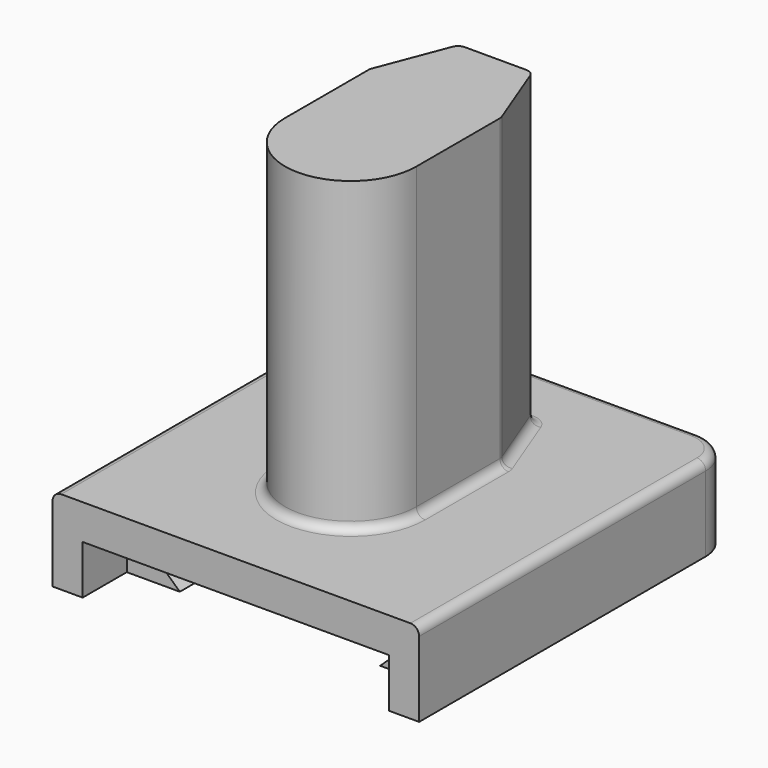
from build123d import *

# Parameters (mm, degrees)
F1_DEPTH = 2.4
F3_DEPTH = 17.61
F5_DEPTH = 2.8
F7_DEPTH = 16.06
F8_R     = 0.5


with BuildPart() as f1:
    # F0 (on Top) → F1 (new body, symmetric)
    with BuildSketch(Plane.XY):
        with BuildLine():
            ThreePointArc((10.47, 9.23), (9.8842135624, 10.6442135624), (8.47, 11.23))
            Line((8.47, 11.23), (-8.47, 11.23))
            ThreePointArc((-8.47, 11.23), (-9.8842135624, 10.6442135624), (-10.47, 9.23))
            Line((-10.47, 9.23), (-10.47, -11.23))
            Line((-10.47, -11.23), (10.47, -11.23))
            Line((10.47, -11.23), (10.47, 9.23))
        make_face()
    extrude(amount=F1_DEPTH, both=True)

    # F2 (on face) → F3 (join)
    with BuildSketch(Plane.XY.offset(2.4)):
        with BuildLine():
            ThreePointArc((-3.75, -3.025), (0, -6.775), (3.75, -3.025))
            Line((3.75, -3.025), (3.75, 3.025))
            Line((3.75, 3.025), (2.1, 7.325))
            Line((2.1, 7.325), (-2.1, 7.325))
            Line((-2.1, 7.325), (-3.75, 3.025))
            Line((-3.75, 3.025), (-3.75, -3.025))
        make_face()
    extrude(amount=F3_DEPTH)

    # F4 (on face) → F5 (cut)
    with BuildSketch(Plane(origin=(0, 0, -2.4), x_dir=(1, 0, 0), z_dir=(0, 0, -1))):
        Polygon((-5.72, 8.08), (-5.72, -7.98), (5.72, -7.98), (5.72, 8.08), (8.75, 8.08), (8.75, 11.23), (-8.75, 11.23), (-8.75, 8.08), align=None)
    extrude(amount=-F5_DEPTH, mode=Mode.SUBTRACT)

    # F6 (on face) → F7 (cut, through all)
    with BuildSketch(Plane.XZ.offset(8.08)):
        Polygon((-8.75, 0.4), (-5.72, -2.4), (-5.72, 0.4), align=None)
        Polygon((5.72, -2.4), (8.75, 0.4), (5.72, 0.4), align=None)
    extrude(amount=-F7_DEPTH, mode=Mode.SUBTRACT)

    # F8
    f8_edges = [f1.edges().sort_by_distance(p)[0] for p in [
        (10.47, -1, 2.4),
        (3.75, 3.025, 11.205),
        (-3.75, 3.025, 11.205),
        (-2.1, 7.325, 11.205),
        (2.1, 7.325, 11.205),
        (0, -6.775, 2.4),
        (9.884214, 10.644214, 2.4),
        (-10.47, -1, 2.4),
        (-9.884214, 10.644214, 2.4),
        (0, 11.23, 2.4),
        (3.75, 0, 2.4),
        (2.925, 5.175, 2.4),
        (0, 7.325, 2.4),
        (-2.925, 5.175, 2.4),
        (-3.75, 0, 2.4),
    ]]
    fillet(f8_edges, radius=F8_R)


solid = f1.part
